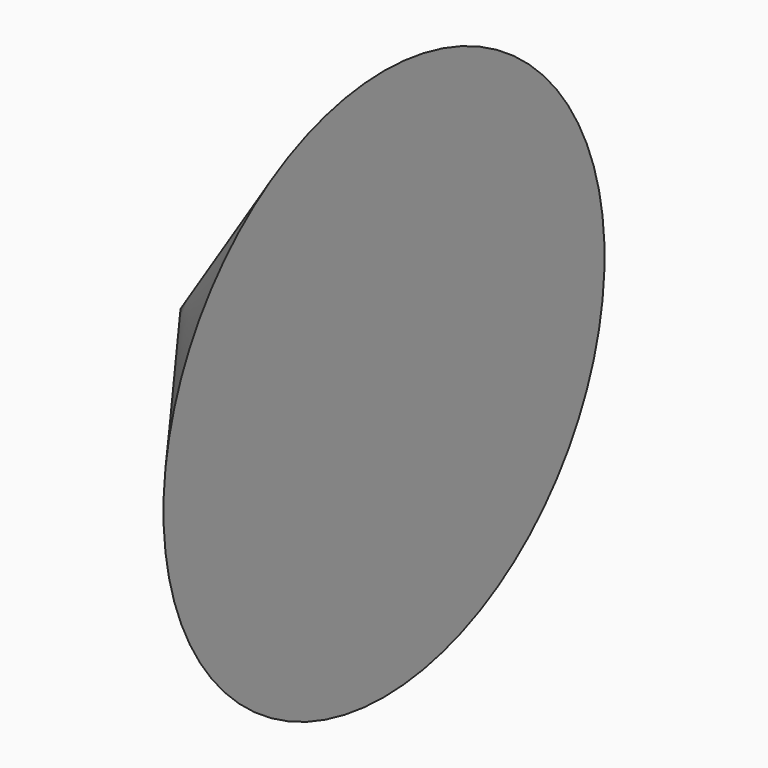
from build123d import *


# Not quite as in the source:
# - the program builds the solid bodies; features that only make, move or delete a surface that nothing else refers to are left out


with BuildPart() as f1:
    # F0 (on Front) → F1 (revolve)
    with BuildSketch(Plane.XZ):
        Polygon((0, 0), (0, 56.1360493302), (-41.4324477315, 0), align=None)
    revolve(axis=Axis((-20.7162238657, 0, 0), (1, 0, 0)))


solid = f1.part
